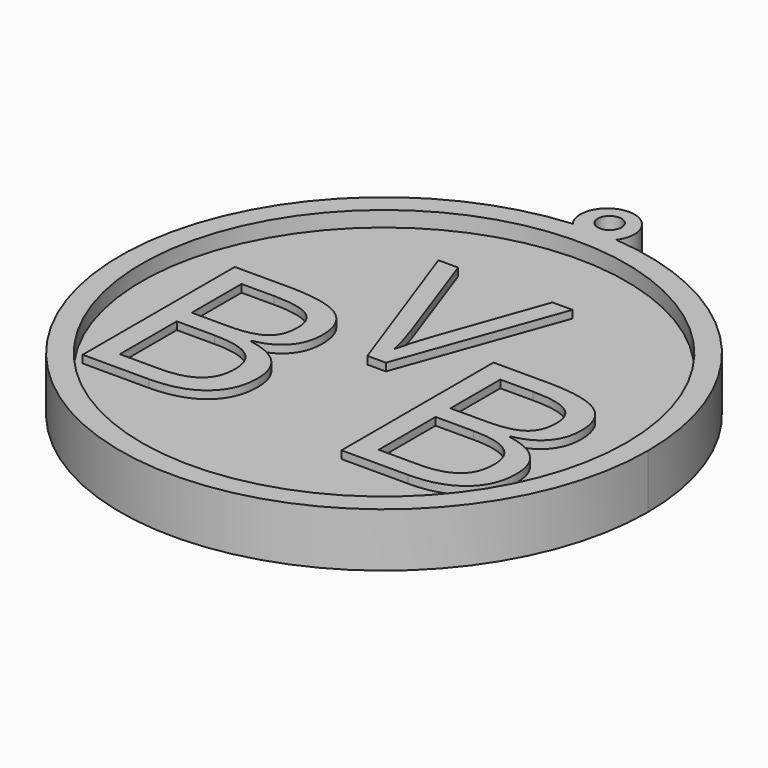
from build123d import *

# Parameters (mm, degrees)
F0_R           = 31.3999463315
F1_DEPTH       = 7
F2_DEPTH       = 5
F3_TEXT_SIZE   = 34.4947012814
F3_TEXT_SIZE_2 = 29.1987719729
F4_DEPTH       = 6
F5_R           = 1.54345
F6_DEPTH       = 20.6


# Not quite as in the source:
# - Text() gives the source's letters only with a copy of the font that has no kerning and outlines rounded to 1/6400 em; it was checked with that copy


with BuildPart() as f1:
    # F0 (on Top) → F1 (new body)
    with BuildSketch(Plane.XY):
        with BuildLine():
            ThreePointArc((-2.8119258593, 34.0826074733), (-23.1664377224, -25.1564548868), (34.1984072615, 0))
            ThreePointArc((34.1984072615, 0), (25.1564548868, 23.1664377224), (2.8119258593, 34.0826074733))
            ThreePointArc((2.8119258593, 34.0826074733), (0, 34.1984072615), (-2.8119258593, 34.0826074733))
        make_face()
        Circle(F0_R, mode=Mode.SUBTRACT)
        with BuildLine():
            ThreePointArc((-2.8119258593, 34.0826074733), (0, 34.1984072615), (2.8119258593, 34.0826074733))
            ThreePointArc((2.8119258593, 34.0826074733), (0, 39.6821750961), (-2.8119258593, 34.0826074733))
        make_face()
    extrude(amount=F1_DEPTH)

    # F0 (on Top) → F2 (join)
    with BuildSketch(Plane.XY):
        Circle(F0_R)
    extrude(amount=F2_DEPTH)

    # F3 (on Top) → F4 (join)
    with BuildSketch(Plane.XY):
        with Locations((-28.1932023354, -17.7959259599)):
            Text('B', F3_TEXT_SIZE, font='Open Sans', text_align=(TextAlign.LEFT, TextAlign.BOTTOM))
        with Locations((5.3386001382, -17.7959259599)):
            Text('B', F3_TEXT_SIZE, font='Open Sans', text_align=(TextAlign.LEFT, TextAlign.BOTTOM))
        with Locations((-9.6355947511, 0)):
            Text('V', F3_TEXT_SIZE_2, font='Open Sans', text_align=(TextAlign.LEFT, TextAlign.BOTTOM))
    extrude(amount=F4_DEPTH)

    # F5 (on Top) → F6 (cut)
    with BuildSketch(Plane.XY):
        with Locations((0, 36.543533206)):
            Circle(F5_R)
    extrude(amount=F6_DEPTH, mode=Mode.SUBTRACT)


solid = f1.part
